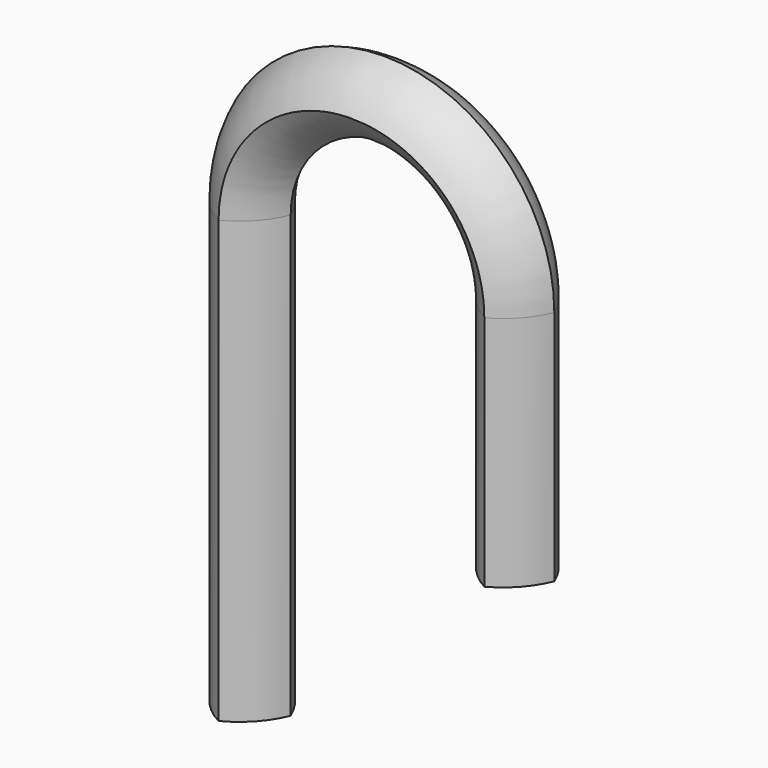
from build123d import *

# Parameters (mm, degrees)
F0_W         = 5.3462936
F0_H         = 14.732
F0_W_2       = 5.5306468
F0_H_2       = 12.7
F1_DEPTH     = 6.35
F2_T1_DEPTH  = 27.432
F2_T3_DEPTH  = 40.132
F2_T6_ANGLE  = 180
F2_T8_ANGLE  = 180
F2_T10_ANGLE = 180
F2_T12_ANGLE = 180


# Not quite as in the source:
# - a fillet or chamfer that OpenCascade refuses, or shapes differently, is made with other operations: its cross-section is extruded or revolved along the edge and cut away or added


with BuildPart() as f1:
    # F0 (on Front) → F1 (new body)
    with BuildSketch(Plane.XZ):
        with BuildLine():
            Line((-2.9891021488, 14.732), (-2.9891021488, 0))
            Line((-2.9891021488, 0), (2.5415446512, 0))
            Line((2.5415446512, 0), (2.5415446512, 14.732))
            ThreePointArc((2.5415446512, 14.732), (8.0721914512, 20.2626468), (13.6028382512, 14.732))
            Line((13.6028382512, 14.732), (18.9491318512, 14.732))
            ThreePointArc((18.9491318512, 14.732), (7.9800148512, 25.701117), (-2.9891021488, 14.732))
        make_face()
        with Locations((16.2759850512, 7.366)):
            Rectangle(F0_W, F0_H)
        with Locations((-0.2237787488, -6.35)):
            Rectangle(F0_W_2, F0_H_2)
    extrude(amount=F1_DEPTH)

    # F2: fillet of radius 5.08 on 4 edges, made by hand

    # F2_s2 → F2_t1 (cut)
    with BuildSketch(Plane.XY.offset(-12.7)):
        with BuildLine():
            ThreePointArc((18.9491318512, -5.08), (17.4612342996, -1.4878975516), (13.8691318512, 0))
            Line((13.8691318512, 0), (18.9491318512, 0))
            Line((18.9491318512, 0), (18.9491318512, -5.08))
        make_face()
        with BuildLine():
            ThreePointArc((13.6028382512, -5.08), (15.0907358028, -1.4878975516), (18.6828382512, 0))
            Line((18.6828382512, 0), (13.6028382512, 0))
            Line((13.6028382512, 0), (13.6028382512, -5.08))
        make_face()
        with BuildLine():
            ThreePointArc((13.6028382512, -1.27), (15.0907358028, -4.8621024484), (18.6828382512, -6.35))
            Line((18.6828382512, -6.35), (13.6028382512, -6.35))
            Line((13.6028382512, -6.35), (13.6028382512, -1.27))
        make_face()
        with BuildLine():
            ThreePointArc((18.9491318512, -1.27), (17.4612342996, -4.8621024484), (13.8691318512, -6.35))
            Line((13.8691318512, -6.35), (18.9491318512, -6.35))
            Line((18.9491318512, -6.35), (18.9491318512, -1.27))
        make_face()
    extrude(amount=F2_T1_DEPTH, mode=Mode.SUBTRACT)

    # F2_s4 → F2_t3 (cut)
    with BuildSketch(Plane.XY.offset(-25.4)):
        with BuildLine():
            ThreePointArc((2.5415446512, -1.27), (1.0536470996, -4.8621024484), (-2.5384553488, -6.35))
            Line((-2.5384553488, -6.35), (2.5415446512, -6.35))
            Line((2.5415446512, -6.35), (2.5415446512, -1.27))
        make_face()
        with BuildLine():
            ThreePointArc((2.5415446512, -5.08), (1.0536470996, -1.4878975516), (-2.5384553488, 0))
            Line((-2.5384553488, 0), (2.5415446512, 0))
            Line((2.5415446512, 0), (2.5415446512, -5.08))
        make_face()
        with BuildLine():
            ThreePointArc((-2.9891021488, -5.08), (-1.5012045972, -1.4878975516), (2.0908978512, 0))
            Line((2.0908978512, 0), (-2.9891021488, 0))
            Line((-2.9891021488, 0), (-2.9891021488, -5.08))
        make_face()
        with BuildLine():
            ThreePointArc((-2.9891021488, -1.27), (-1.5012045972, -4.8621024484), (2.0908978512, -6.35))
            Line((2.0908978512, -6.35), (-2.9891021488, -6.35))
            Line((-2.9891021488, -6.35), (-2.9891021488, -1.27))
        make_face()
    extrude(amount=F2_T3_DEPTH, mode=Mode.SUBTRACT)

    # F2_s5 → F2_t6 (revolve, cut)
    with BuildSketch(Plane.XY.offset(14.732)):
        with BuildLine():
            ThreePointArc((18.9491318512, -1.27), (17.4612342996, -4.8621024484), (13.8691318512, -6.35))
            Line((13.8691318512, -6.35), (18.9491318512, -6.35))
            Line((18.9491318512, -6.35), (18.9491318512, -1.27))
        make_face()
    revolve(axis=Axis((7.9800148512, -6.35, 14.732), (0, -1, 0)), revolution_arc=F2_T6_ANGLE, mode=Mode.SUBTRACT)

    # F2_s7 → F2_t8 (revolve, cut)
    with BuildSketch(Plane.XY.offset(14.732)):
        with BuildLine():
            ThreePointArc((2.5415446512, -5.08), (1.0536470996, -1.4878975516), (-2.5384553488, 0))
            Line((-2.5384553488, 0), (2.5415446512, 0))
            Line((2.5415446512, 0), (2.5415446512, -5.08))
        make_face()
    revolve(axis=Axis((8.0721914512, 0, 14.732), (0, 1, 0)), revolution_arc=F2_T8_ANGLE, mode=Mode.SUBTRACT)

    # F2_s9 → F2_t10 (revolve, cut)
    with BuildSketch(Plane.XY.offset(14.732)):
        with BuildLine():
            ThreePointArc((2.5415446512, -1.27), (1.0536470996, -4.8621024484), (-2.5384553488, -6.35))
            Line((-2.5384553488, -6.35), (2.5415446512, -6.35))
            Line((2.5415446512, -6.35), (2.5415446512, -1.27))
        make_face()
    revolve(axis=Axis((8.0721914512, -6.35, 14.732), (0, 1, 0)), revolution_arc=F2_T10_ANGLE, mode=Mode.SUBTRACT)

    # F2_s11 → F2_t12 (revolve, cut)
    with BuildSketch(Plane.XY.offset(14.732)):
        with BuildLine():
            ThreePointArc((18.9491318512, -5.08), (17.4612342996, -1.4878975516), (13.8691318512, 0))
            Line((13.8691318512, 0), (18.9491318512, 0))
            Line((18.9491318512, 0), (18.9491318512, -5.08))
        make_face()
    revolve(axis=Axis((7.9800148512, 0, 14.732), (0, -1, 0)), revolution_arc=F2_T12_ANGLE, mode=Mode.SUBTRACT)


solid = f1.part
